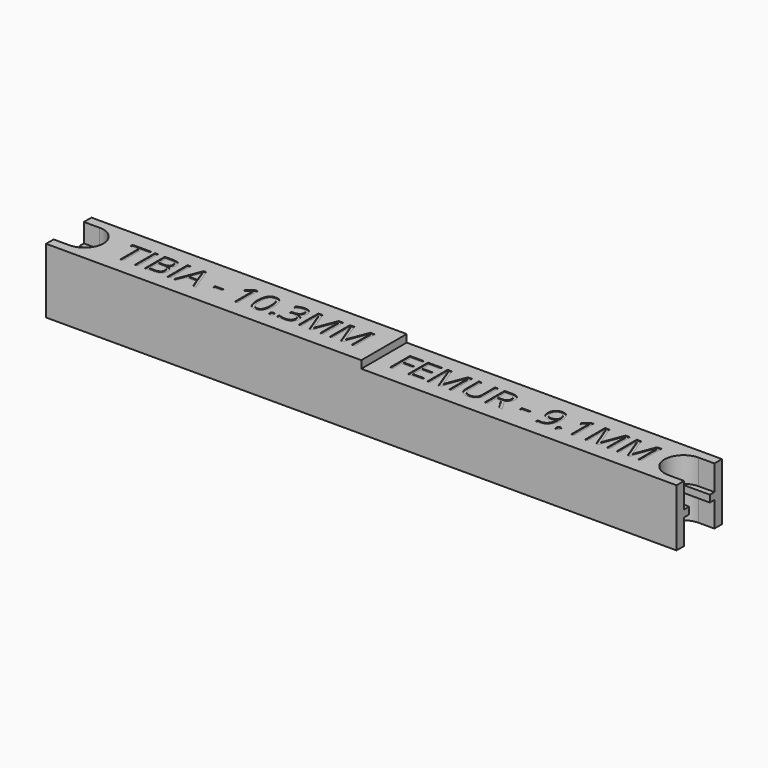
from build123d import *

# Parameters (mm, degrees)
F1_DEPTH      = 9
F4_DEPTH      = 3
F5_DEPTH      = 4
F7_DEPTH      = 6
F9_DEPTH      = 4
F11_DEPTH     = 2
F13_DEPTH     = 2
F14_TEXT_SIZE = 5.5555555556
F16_DEPTH     = 0.1
F15_TEXT_SIZE = 5.5555555556
F17_DEPTH     = 0.1
F18_TEXT_SIZE = 5.5555555556
F19_DEPTH     = 0.1


# Not quite as in the source:
# - Text() gives the source's letters only with a copy of the font that has no kerning and outlines rounded to 1/6400 em; it was checked with that copy


with BuildPart() as f1:
    # F0 (on Front) → F1 (new body)
    with BuildSketch(Plane.XZ):
        Polygon((0, 10.3), (0, 0), (50, 0), (100, 0), (100, 9.1), (50, 9.1), (50, 10.3), align=None)
    extrude(amount=F1_DEPTH)

    # F2 (on face) → F4 (cut)
    with BuildSketch(Plane.XY.offset(10.3)):
        with BuildLine():
            Line((2.5, -1.5), (0, -1.5))
            Line((0, -1.5), (0, -4.5))
            Line((0, -4.5), (0, -7.5))
            Line((0, -7.5), (2.5, -7.5))
            ThreePointArc((2.5, -7.5), (5.5, -4.5), (2.5, -1.5))
        make_face()
    extrude(amount=-F4_DEPTH, mode=Mode.SUBTRACT)

    # F3 (on face) → F5 (cut)
    with BuildSketch(Plane.XY.offset(9.1)):
        with BuildLine():
            Line((100, -4.5), (100, -1.5))
            Line((100, -1.5), (97.5, -1.5))
            ThreePointArc((97.5, -1.5), (94.5, -4.5), (97.5, -7.5))
            Line((97.5, -7.5), (100, -7.5))
            Line((100, -7.5), (100, -4.5))
        make_face()
    extrude(amount=-F5_DEPTH, mode=Mode.SUBTRACT)

    # F6 (on face) → F7 (cut)
    with BuildSketch(Plane(origin=(0, 0, 0), x_dir=(1, 0, 0), z_dir=(0, 0, -1))):
        with BuildLine():
            Line((2.5, 7.5), (0, 7.5))
            Line((0, 7.5), (0, 4.5))
            Line((0, 4.5), (0, 1.5))
            Line((0, 1.5), (2.5, 1.5))
            ThreePointArc((2.5, 1.5), (5.5, 4.5), (2.5, 7.5))
        make_face()
    extrude(amount=-F7_DEPTH, mode=Mode.SUBTRACT)

    # F8 (on face) → F9 (cut)
    with BuildSketch(Plane(origin=(0, 0, 0), x_dir=(1, 0, 0), z_dir=(0, 0, -1))):
        with BuildLine():
            Line((100, 4.5), (100, 7.5))
            Line((100, 7.5), (97.5, 7.5))
            ThreePointArc((97.5, 7.5), (94.5, 4.5), (97.5, 1.5))
            Line((97.5, 1.5), (100, 1.5))
            Line((100, 1.5), (100, 4.5))
        make_face()
    extrude(amount=-F9_DEPTH, mode=Mode.SUBTRACT)

    # F10 (on face) → F11 (cut)
    with BuildSketch(Plane.XY.offset(7.3)):
        with BuildLine():
            Line((0, -2.4), (0, -6.5))
            Line((0, -6.5), (4.7360679775, -6.5))
            ThreePointArc((4.7360679775, -6.5), (5.4992178836, -4.4315011927), (4.6424285286, -2.4))
            Line((4.6424285286, -2.4), (0, -2.4))
        make_face()
    extrude(amount=-F11_DEPTH, mode=Mode.SUBTRACT)

    # F12 (on face) → F13 (cut)
    with BuildSketch(Plane(origin=(0, 0, 4), x_dir=(1, 0, 0), z_dir=(0, 0, -1))):
        with BuildLine():
            Line((100, 2.4), (100, 6.5))
            Line((100, 6.5), (95.2639320225, 6.5))
            ThreePointArc((95.2639320225, 6.5), (94.5007821164, 4.4315011927), (95.3575714714, 2.4))
            Line((95.3575714714, 2.4), (100, 2.4))
        make_face()
    extrude(amount=-F13_DEPTH, mode=Mode.SUBTRACT)

    # F14 (on face) → F16 (cut)
    with BuildSketch(Plane.XY.offset(10.3)):
        with Locations((8.5, -6.5)):
            Text('TIBIA - 10.3MM', F14_TEXT_SIZE, font='Open Sans', text_align=(TextAlign.LEFT, TextAlign.BOTTOM))
    extrude(amount=-F16_DEPTH, mode=Mode.SUBTRACT)

    # F15 (on face) → F17 (cut)
    with BuildSketch(Plane.XY.offset(9.1)):
        with Locations((52, -6.5)):
            Text('FEMUR - 9.1MM', F15_TEXT_SIZE, font='Open Sans', text_align=(TextAlign.LEFT, TextAlign.BOTTOM))
    extrude(amount=-F17_DEPTH, mode=Mode.SUBTRACT)

    # F18 (on face) → F19 (cut)
    with BuildSketch(Plane(origin=(0, 0, 0), x_dir=(1, 0, 0), z_dir=(0, 0, -1))):
        with Locations((11.4265847951, 2.5)):
            Text('FLEX PLI CABLE SPACER TOOL', F18_TEXT_SIZE, font='Open Sans', text_align=(TextAlign.LEFT, TextAlign.BOTTOM))
    extrude(amount=-F19_DEPTH, mode=Mode.SUBTRACT)


solid = f1.part
